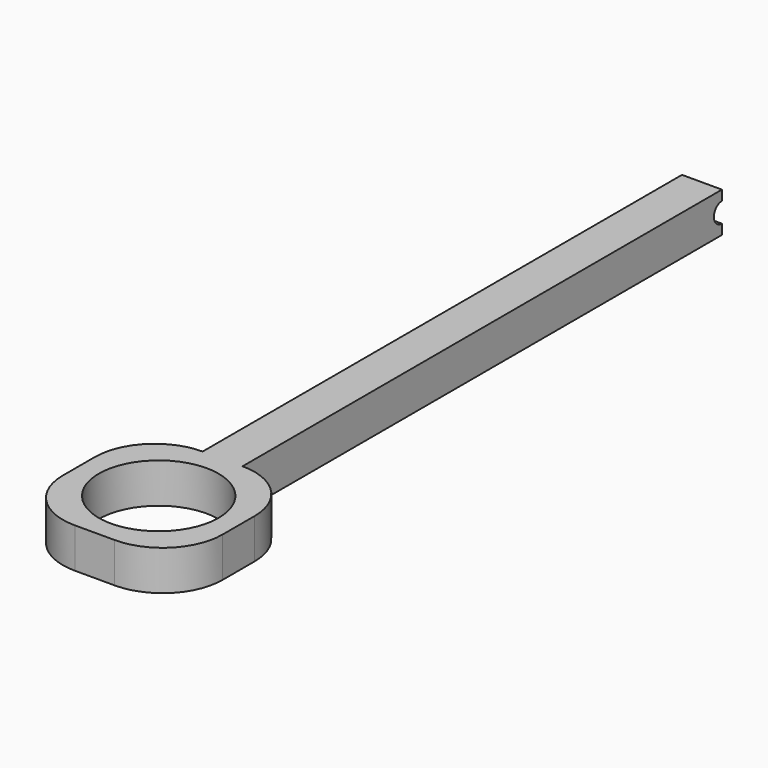
from build123d import *

# Parameters (mm, degrees)
F0_W     = 12.7
F0_H     = 12.7
F1_DEPTH = 190.5
F2_W     = 50.8
F2_H     = 50.8
F3_DEPTH = 12.7
F4_R     = 19.05
F5_DEPTH = 12.701
F6_R     = 19.04999
F7_R     = 3.175
F8_DEPTH = 31.751


# Not quite as in the source:
# - a fillet or chamfer is up to 0.001 mm smaller than in the source, because OpenCascade refuses the exact size


with BuildPart() as f1:
    # F0 (on Front) → F1 (new body)
    with BuildSketch(Plane.XZ):
        with Locations((6.35, -6.35)):
            Rectangle(F0_W, F0_H)
    extrude(amount=F1_DEPTH)

    # F2 (on face) → F3 (join)
    with BuildSketch(Plane.XY):
        with Locations((6.35, -215.9)):
            Rectangle(F2_W, F2_H)
    extrude(amount=-F3_DEPTH)

    # F4 (on face) → F5 (cut, through all)
    with BuildSketch(Plane.XY):
        with Locations((6.35, -215.9)):
            Circle(F4_R)
    extrude(amount=-F5_DEPTH, mode=Mode.SUBTRACT)

    # F6 (radius 19.05 in the source; OpenCascade refuses exactly that, so slightly less here)
    f6_edges = [f1.edges().sort_by_distance(p)[0] for p in [
        (31.75, -241.3, -6.35),
        (31.75, -190.5, -6.35),
        (-19.05, -241.3, -6.35),
        (-19.05, -190.5, -6.35),
    ]]
    fillet(f6_edges, radius=F6_R)

    # F7 (on face) → F8 (cut, through all)
    with BuildSketch(Plane.YZ.offset(12.7)):
        with Locations((0, -6.35)):
            Circle(F7_R)
    extrude(amount=-F8_DEPTH, mode=Mode.SUBTRACT)


solid = f1.part
